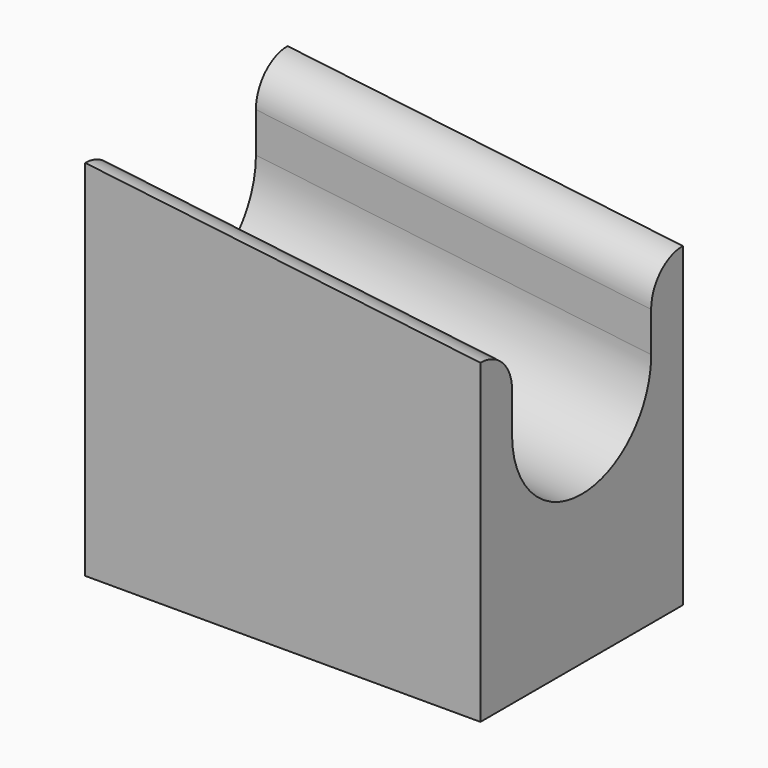
from build123d import *

# Parameters (mm, degrees)
F1_DEPTH = 32
F4_DEPTH = 55
F5_R     = 4.99999


# Not quite as in the source:
# - a fillet or chamfer is up to 0.001 mm smaller than in the source, because OpenCascade refuses the exact size


with BuildPart() as f1:
    # F0 (on Front) → F1 (new body)
    with BuildSketch(Plane.XZ):
        Polygon((0, 46), (0, 0), (50, 0), (50, 40), align=None)
    extrude(amount=-F1_DEPTH)

    # F3 (on face) → F4 (cut, symmetric)
    with BuildSketch(Plane(origin=(44.5961827524, 0, -5.3177728391), x_dir=(0, 1, 0), z_dir=(0.9929655081, 0, -0.1184039683))):
        with BuildLine():
            Line((5, 47.6340688765), (5, 35.6388187396))
            ThreePointArc((5, 35.6388187396), (16, 24.6388187396), (27, 35.6388187396))
            Line((27, 35.6388187396), (27, 47.6340688765))
            Line((27, 47.6340688765), (5, 47.6340688765))
        make_face()
    extrude(amount=F4_DEPTH, both=True, mode=Mode.SUBTRACT)

    # F5 (radius 5 in the source; OpenCascade refuses exactly that, so slightly less here)
    f5_edges = [f1.edges().sort_by_distance(p)[0] for p in [
        (25, 27, 43),
        (25, 5, 43),
    ]]
    fillet(f5_edges, radius=F5_R)


solid = f1.part
